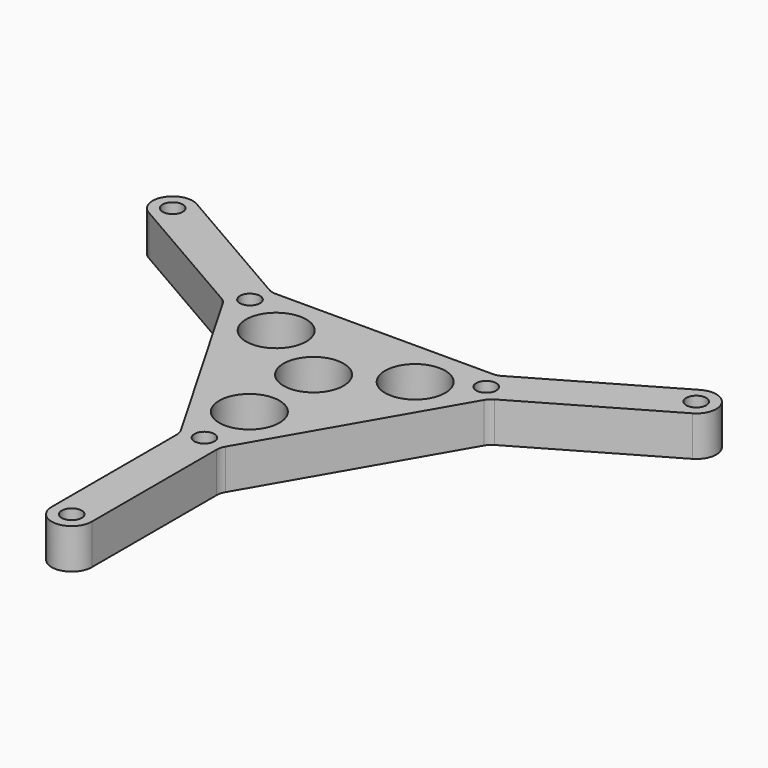
from build123d import *

# Parameters (mm, degrees)
F0_R     = 1.5875
F0_R_2   = 4.7625
F1_DEPTH = 6.35
F2_R     = 2.54


# Not quite as in the source:
# - a length typed as a fraction of an inch, garbled in the dataset ("3 / 203.2 mm" for 3/8 in), is restored


with BuildPart() as f1:
    # F0 (on Top) → F1 (new body)
    with BuildSketch(Plane.XY):
        with BuildLine():
            Line((3.175, -22.440738686), (0, -27.94))
            Line((0, -27.94), (-3.175, -22.440738686))
            Line((-3.175, -22.440738686), (-3.175, -47.840738686))
            ThreePointArc((-3.175, -47.840738686), (0, -51.015738686), (3.175, -47.840738686))
            Line((3.175, -47.840738686), (3.175, -22.440738686))
        make_face()
        with Locations((0, -47.840738686)):
            Circle(F0_R, mode=Mode.SUBTRACT)
        Polygon((-3.175, -22.440738686), (0, -27.94), (3.175, -22.440738686), (21.0217497817, 8.470738686), (24.1967497817, 13.97), (17.8467497817, 13.97), (-17.8467497817, 13.97), (-24.1967497817, 13.97), (-21.0217497817, 8.470738686), align=None)
        with Locations((0, -21.59)):
            Circle(F0_R, mode=Mode.SUBTRACT)
        with Locations((0, -12.7)):
            Circle(F0_R_2, mode=Mode.SUBTRACT)
        Circle(F0_R_2, mode=Mode.SUBTRACT)
        with Locations((-10.9985226281, 6.35)):
            Circle(F0_R_2, mode=Mode.SUBTRACT)
        with Locations((-18.6974884677, 10.795)):
            Circle(F0_R, mode=Mode.SUBTRACT)
        with Locations((10.9985226281, 6.35)):
            Circle(F0_R_2, mode=Mode.SUBTRACT)
        with Locations((18.6974884677, 10.795)):
            Circle(F0_R, mode=Mode.SUBTRACT)
        with BuildLine():
            Line((-43.0187950379, 21.170738686), (-21.0217497817, 8.470738686))
            Line((-21.0217497817, 8.470738686), (-24.1967497817, 13.97))
            Line((-24.1967497817, 13.97), (-17.8467497817, 13.97))
            Line((-17.8467497817, 13.97), (-39.8437950379, 26.67))
            ThreePointArc((-39.8437950379, 26.67), (-44.1809256949, 25.507869343), (-43.0187950379, 21.170738686))
        make_face()
        with Locations((-41.4312950379, 23.920369343)):
            Circle(F0_R, mode=Mode.SUBTRACT)
        with BuildLine():
            Line((24.1967497817, 13.97), (21.0217497817, 8.470738686))
            Line((21.0217497817, 8.470738686), (43.0187950379, 21.170738686))
            ThreePointArc((43.0187950379, 21.170738686), (44.1809256949, 25.507869343), (39.8437950379, 26.67))
            Line((39.8437950379, 26.67), (17.8467497817, 13.97))
            Line((17.8467497817, 13.97), (24.1967497817, 13.97))
        make_face()
        with Locations((41.4312950379, 23.920369343)):
            Circle(F0_R, mode=Mode.SUBTRACT)
    extrude(amount=F1_DEPTH)

    # F2
    f2_edges = [f1.edges().sort_by_distance(p)[0] for p in [
        (-3.175, -22.440739, 3.175),
        (-21.02175, 8.470739, 3.175),
        (-17.84675, 13.97, 3.175),
        (17.84675, 13.97, 3.175),
        (21.02175, 8.470739, 3.175),
        (3.175, -22.440739, 3.175),
    ]]
    fillet(f2_edges, radius=F2_R)


solid = f1.part
